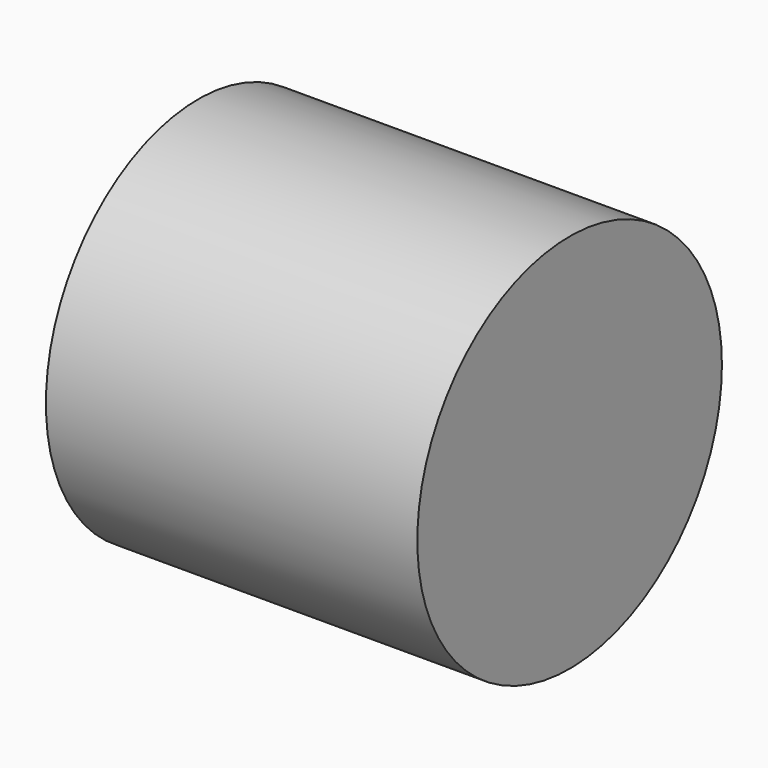
from build123d import *

# Parameters (mm, degrees)
F1_R     = 12.8141976258
F1_R_2   = 10
F2_DEPTH = 25


# Not quite as in the source:
# - the program builds the solid bodies; features that only make, move or delete a surface that nothing else refers to are left out


with BuildPart() as f2:
    # F1 (on face) → F2 (new body)
    with BuildSketch(Plane.YZ):
        with Locations((2.2681457922, 0)):
            Circle(F1_R)
        with Locations((2.0192302763, 0)):
            Circle(F1_R_2, mode=Mode.SUBTRACT)
        with Locations((2.0192302763, 0)):
            Circle(F1_R_2)
    extrude(amount=F2_DEPTH)


solid = f2.part
